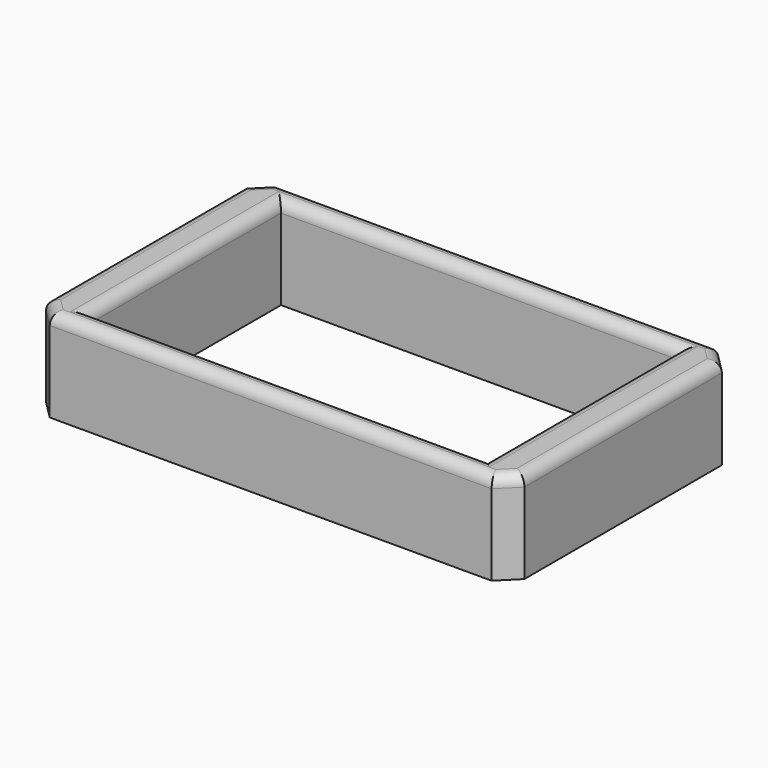
from build123d import *

# Parameters (mm, degrees)
F0_W     = 108
F0_H     = 65
F1_DEPTH = 25
F2_R     = 2.99999


# Not quite as in the source:
# - a fillet or chamfer is up to 0.001 mm smaller than in the source, because OpenCascade refuses the exact size


with BuildPart() as f1:
    # F0 (on Top) → F1 (new body)
    with BuildSketch(Plane.XY):
        Polygon((60.0555262864, 38.5), (-60.0555262864, 38.5), (-65, 33.5555262864), (-65, -33.5555262864), (-60.0555262864, -38.5), (60.0555262864, -38.5), (65, -33.5555262864), (65, 33.5555262864), align=None)
        Rectangle(F0_W, F0_H, mode=Mode.SUBTRACT)
    extrude(amount=F1_DEPTH)

    # F2 (radius 3 in the source; OpenCascade refuses exactly that, so slightly less here)
    f2_edges = [f1.edges().sort_by_distance(p)[0] for p in [
        (65, 0, 25),
        (62.527763, 36.027763, 25),
        (0, 38.5, 25),
        (-62.527763, 36.027763, 25),
        (-65, 0, 25),
        (-62.527763, -36.027763, 25),
        (0, -38.5, 25),
        (62.527763, -36.027763, 25),
        (-54, 0, 25),
        (0, 32.5, 25),
        (54, 0, 25),
        (0, -32.5, 25),
    ]]
    fillet(f2_edges, radius=F2_R)


solid = f1.part
